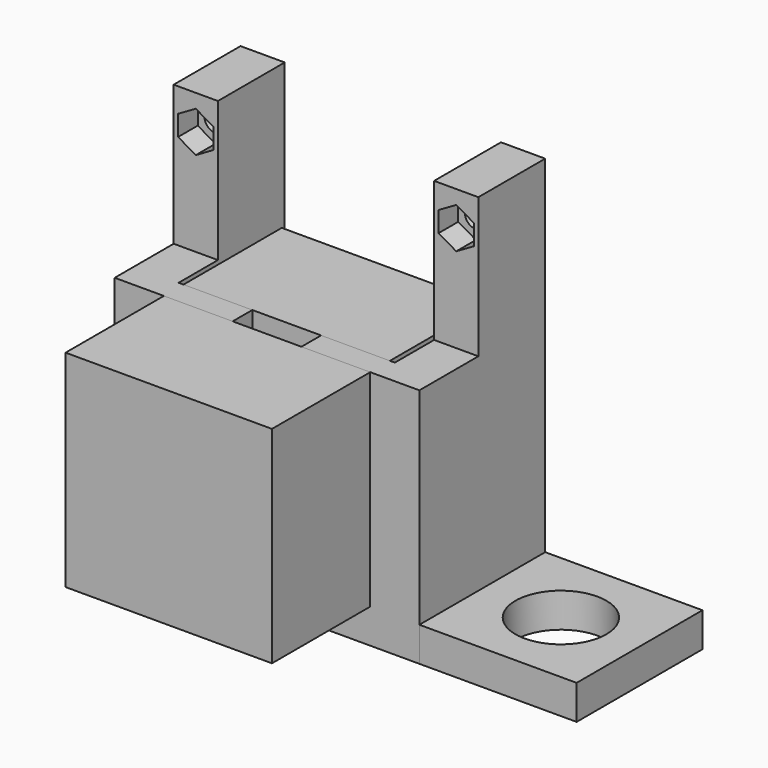
from build123d import *

# Parameters (mm, degrees)
F1_R      = 2.25
F2_DEPTH  = 12
F4_DEPTH  = 5
F5_W      = 44
F5_H      = 10
F5_H_2    = 5
F6_DEPTH  = 7
F7_DEPTH  = 42
F8_R      = 1.7
F8_R_2    = 13
F9_DEPTH  = 5
F11_REACH = 63.8670687473
F12_R     = 1.7
F13_DEPTH = 25
F14_W     = 42
F14_H     = 42
F14_R     = 1.7
F14_R_2   = 13
F15_DEPTH = 25
F16_W     = 32
F16_H     = 32
F16_R     = 9.25
F17_DEPTH = 7


with BuildPart() as f2:
    # F1 (on Front) → F2 (new body)
    with BuildSketch(Plane.XZ):
        Polygon((-27, 56.5), (-36, 56.5), (-36, -21), (26, -21), (26, 56.5), (17, 56.5), (17, -14), (-27, -14), align=None)
        with Locations((-31.5, 49.5)):
            Circle(F1_R, mode=Mode.SUBTRACT)
        with Locations((21.5, 49.5)):
            Circle(F1_R, mode=Mode.SUBTRACT)
    extrude(amount=-F2_DEPTH)

    # F3 (on face) → F4 (join)
    with BuildSketch(Plane.XZ):
        Polygon((-27, -14), (-27, 56.5), (-36, 56.5), (-36, -21), (26, -21), (26, 56.5), (17, 56.5), (17, -14), align=None)
        Polygon((-31.5, 53.6569219382), (-27.9, 51.5784609691), (-27.9, 47.4215390309), (-31.5, 45.3430780618), (-35.1, 47.4215390309), (-35.1, 51.5784609691), align=None, mode=Mode.SUBTRACT)
        Polygon((21.5, 53.6569219382), (25.1, 51.5784609691), (25.1, 47.4215390309), (21.5, 45.3430780618), (17.9, 47.4215390309), (17.9, 51.5784609691), align=None, mode=Mode.SUBTRACT)
    extrude(amount=F4_DEPTH)

    # F5 (on face) → F6 (join, through all)
    with BuildSketch(Plane.XY.offset(-14)):
        with Locations((-5, -10)):
            Rectangle(F5_W, F5_H)
        with Locations((-5, -17.5)):
            Rectangle(F5_W, F5_H_2)
        Polygon((-27, -15), (-27, -5), (-36, -5), (-36, -20), (-27, -20), align=None)
        Polygon((26, -5), (17, -5), (17, -15), (17, -20), (26, -20), align=None)
    extrude(amount=-F6_DEPTH)

    # F5 (on face) → F7 (join)
    with BuildSketch(Plane.XY.offset(-14)):
        with Locations((-5, -17.5)):
            Rectangle(F5_W, F5_H_2)
        Polygon((-27, -15), (-27, -5), (-36, -5), (-36, -20), (-27, -20), align=None)
        Polygon((26, -5), (17, -5), (17, -15), (17, -20), (26, -20), align=None)
    extrude(amount=F7_DEPTH)

    # F8 (on face) → F9 (cut, through all)
    with BuildSketch(Plane.XZ.offset(20)):
        with Locations((-20.5, 22.5)):
            Circle(F8_R)
        with Locations((-5, 7)):
            Circle(F8_R_2)
        with Locations((-20.5, -8.5)):
            Circle(F8_R)
        with Locations((10.5, -8.5)):
            Circle(F8_R)
        with Locations((10.5, 22.5)):
            Circle(F8_R)
    extrude(amount=-F9_DEPTH, mode=Mode.SUBTRACT)

    f11_end = f2.faces().sort_by_distance((-18, -17.5, 7))[0]
    # F10 (on face) → F11 (cut, up to a face of the model that its end follows)
    with BuildSketch(Plane.XY.offset(28)):
        Polygon((2, -15), (-5, -15), (-12, -15), (-12, -20), (2, -20), align=None)
    f11_long = extrude(amount=-F11_REACH, mode=Mode.PRIVATE)
    add(split(f11_long, bisect_by=f11_end, keep=Keep.ALL, mode=Mode.PRIVATE).solids().sort_by_distance((-5, -17.5, 28))[0], mode=Mode.SUBTRACT)


with BuildPart() as f13:
    # F12 (on face) → F13 (new body)
    with BuildSketch(Plane(origin=(0, -15, 0), x_dir=(-1, 0, 0), z_dir=(0, 1, 0))):
        with BuildLine():
            Line((-16, -14), (26, -14))
            Line((26, -14), (26, 28))
            Line((26, 28), (12, 28))
            Line((12, 28), (12, 17.9544511501))
            ThreePointArc((12, 17.9544511501), (5, -6), (-2, 17.9544511501))
            Line((-2, 17.9544511501), (-2, 28))
            Line((-2, 28), (-16, 28))
            Line((-16, 28), (-16, -14))
        make_face()
        with Locations((-10.5, -8.5)):
            Circle(F12_R, mode=Mode.SUBTRACT)
        with Locations((20.5, -8.5)):
            Circle(F12_R, mode=Mode.SUBTRACT)
        with Locations((-10.5, 22.5)):
            Circle(F12_R, mode=Mode.SUBTRACT)
        with Locations((20.5, 22.5)):
            Circle(F12_R, mode=Mode.SUBTRACT)
        with BuildLine():
            Line((12, 17.9544511501), (12, 28))
            Line((12, 28), (-2, 28))
            Line((-2, 28), (-2, 17.9544511501))
            ThreePointArc((-2, 17.9544511501), (5, -6), (12, 17.9544511501))
        make_face()
        with Locations((-10.5, 22.5)):
            Circle(F12_R)
        with Locations((20.5, 22.5)):
            Circle(F12_R)
        with Locations((-10.5, -8.5)):
            Circle(F12_R)
        with Locations((20.5, -8.5)):
            Circle(F12_R)
    extrude(amount=F13_DEPTH)


with BuildPart() as f15:
    # F14 (on face) → F15 (new body)
    with BuildSketch(Plane.XZ.offset(20)):
        with Locations((-5, 7)):
            Rectangle(F14_W, F14_H)
        with Locations((-20.5, -8.5)):
            Circle(F14_R, mode=Mode.SUBTRACT)
        with Locations((10.5, -8.5)):
            Circle(F14_R, mode=Mode.SUBTRACT)
        with Locations((-20.5, 22.5)):
            Circle(F14_R, mode=Mode.SUBTRACT)
        with Locations((-5, 7)):
            Circle(F14_R_2, mode=Mode.SUBTRACT)
        with Locations((10.5, 22.5)):
            Circle(F14_R, mode=Mode.SUBTRACT)
    extrude(amount=F15_DEPTH)

    # F8 (on face) → F15, piece 2 (join)
    with BuildSketch(Plane.XZ.offset(20)):
        with Locations((-20.5, 22.5)):
            Circle(F8_R)
    extrude(amount=F15_DEPTH)

    # F8 (on face) → F15, piece 3 (join)
    with BuildSketch(Plane.XZ.offset(20)):
        with Locations((-5, 7)):
            Circle(F8_R_2)
    extrude(amount=F15_DEPTH)

    # F8 (on face) → F15, piece 4 (join)
    with BuildSketch(Plane.XZ.offset(20)):
        with Locations((-20.5, -8.5)):
            Circle(F8_R)
    extrude(amount=F15_DEPTH)

    # F8 (on face) → F15, piece 5 (join)
    with BuildSketch(Plane.XZ.offset(20)):
        with Locations((10.5, 22.5)):
            Circle(F8_R)
    extrude(amount=F15_DEPTH)

    # F8 (on face) → F15, piece 6 (join)
    with BuildSketch(Plane.XZ.offset(20)):
        with Locations((10.5, -8.5)):
            Circle(F8_R)
    extrude(amount=F15_DEPTH)


with BuildPart() as f17:
    # F16 (on face) → F17 (new body, through all)
    with BuildSketch(Plane(origin=(0, 0, -21), x_dir=(1, 0, 0), z_dir=(0, 0, -1))):
        with Locations((42, 4)):
            Rectangle(F16_W, F16_H)
        with Locations((42, 4)):
            Circle(F16_R, mode=Mode.SUBTRACT)
    extrude(amount=-F17_DEPTH)


solid = Compound([f2.part, f13.part, f15.part, f17.part])
